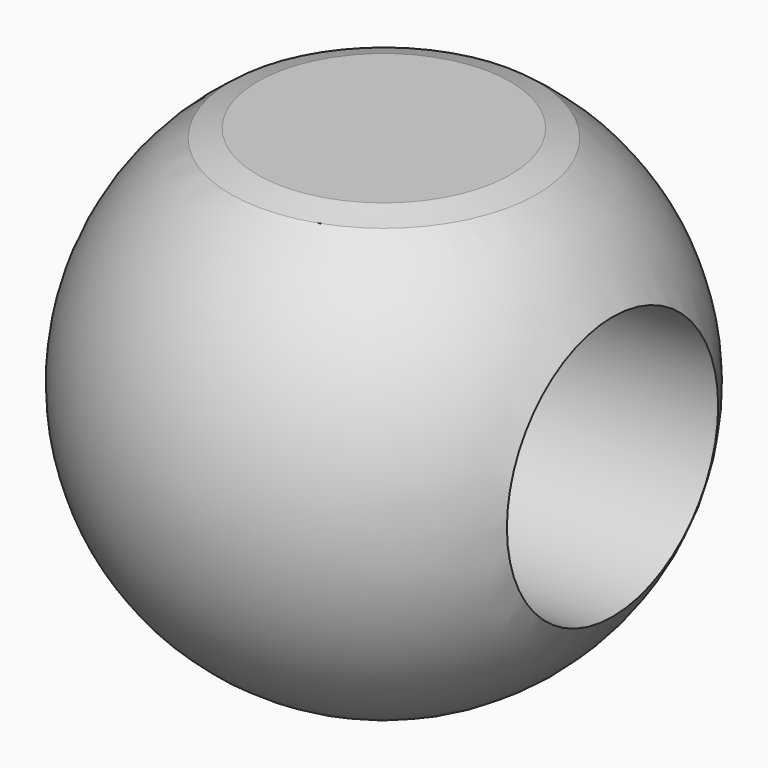
from build123d import *

# Parameters (mm, degrees)
F2_R     = 20
F3_DEPTH = 50
F4_W     = 62.4089296907
F4_H     = 39.0701051801
F5_DEPTH = 50


# Not quite as in the source:
# - a fillet or chamfer that OpenCascade refuses, or shapes differently, is made with other operations: its cross-section is extruded or revolved along the edge and cut away or added


with BuildPart() as f1:
    # F0 (on Top) → F1 (revolve)
    with BuildSketch(Plane.XY):
        with BuildLine():
            Line((0, 40), (0, -40))
            ThreePointArc((0, -40), (40, 0), (0, 40))
        make_face()
    revolve(axis=Axis((0, 0, 0), (0, -1, 0)))

    # F2 (on Right) → F3 (cut, symmetric)
    with BuildSketch(Plane.YZ):
        Circle(F2_R)
    extrude(amount=F3_DEPTH, both=True, mode=Mode.SUBTRACT)

    # F4 (on Right) → F5 (cut, symmetric)
    with BuildSketch(Plane.YZ):
        with Locations((0.7427642122, 53.4269148484)):
            Rectangle(F4_W, F4_H)
    extrude(amount=F5_DEPTH, both=True, mode=Mode.SUBTRACT)

    # F6: chamfer of 2 on 1 edges, made by hand

    # F6_s1 → F6_t2 (revolve, cut)
    with BuildSketch(Plane.YZ):
        with BuildLine():
            Line((23.2462048843, 32.5816827787), (19.0643837553, 33.916183436))
            Line((19.0643837553, 33.916183436), (19.0643837553, 33.956183436))
            ThreePointArc((19.0643837553, 33.956183436), (20.1545935913, 33.9318622583), (21.2448034273, 33.9318622583))
            Line((21.2448034273, 33.9318622583), (21.2660482307, 33.9257541206))
            ThreePointArc((21.2660482307, 33.9257541206), (22.2709130322, 33.2747356521), (23.2693748758, 32.6142887827))
            Line((23.2693748758, 32.6142887827), (23.2462048843, 32.5816827787))
        make_face()
    revolve(axis=Axis((0, 0, 33.8918622583), (0, 0, -1)), mode=Mode.SUBTRACT)


solid = f1.part
